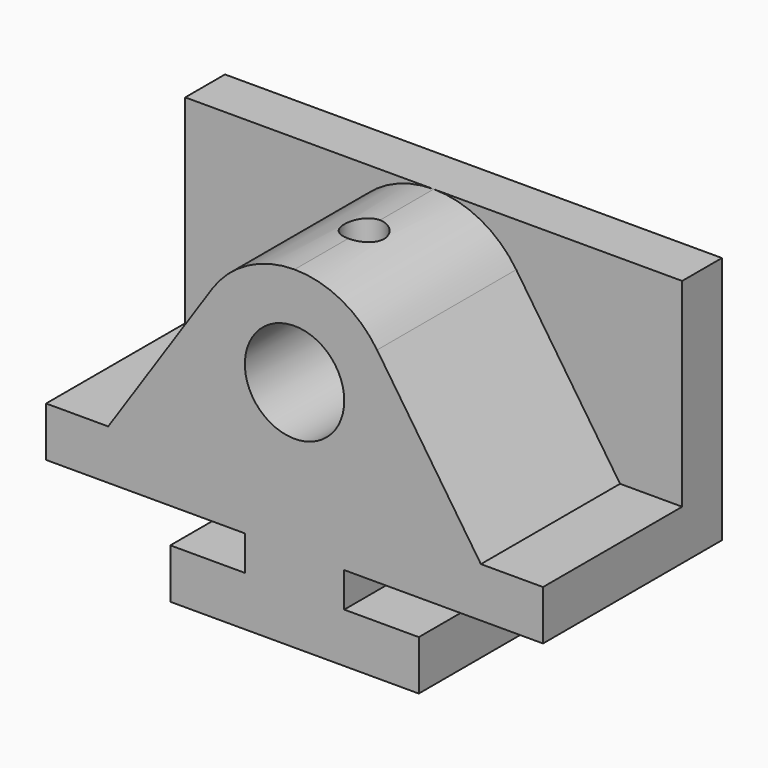
from build123d import *
from build123d import SkipClean  # not in build123d's __all__

# Parameters (mm, degrees)
F0_W     = 127
F0_H     = 85.09
F1_DEPTH = 57.15
F3_DEPTH = 57.151
F4_DEPTH = 44.45
F5_R     = 12.7
F6_DEPTH = 44.45
F7_R     = 5.08
F8_DEPTH = 13.7612578348


with BuildPart() as f1:
    # F0 (on Front) → F1 (new body)
    with BuildSketch(Plane.XZ):
        with Locations((63.5, 42.545)):
            Rectangle(F0_W, F0_H)
    extrude(amount=F1_DEPTH)

    # F2 (on face) → F3 (cut, through all)
    with BuildSketch(Plane.XZ.offset(57.15)):
        Polygon((0, 0), (31.75, 0), (31.75, 12.7), (50.8, 12.7), (50.8, 21.59), (0, 21.59), align=None)
        Polygon((95.25, 12.7), (95.25, 0), (127, 0), (127, 21.59), (76.2, 21.59), (76.2, 12.7), align=None)
    extrude(amount=-F3_DEPTH, mode=Mode.SUBTRACT)

    # F2 (on face) → F4 (cut)
    with BuildSketch(Plane.XZ.offset(57.15)):
        with BuildLine():
            Line((0, 85.09), (0, 34.29))
            Line((0, 34.29), (15.875, 34.29))
            Line((15.875, 34.29), (42.4065743945, 73.8401730104))
            ThreePointArc((42.4065743945, 73.8401730104), (51.5470588235, 82.1017647059), (63.5, 85.09))
            Line((63.5, 85.09), (0, 85.09))
        make_face()
        with BuildLine():
            Line((111.125, 34.29), (127, 34.29))
            Line((127, 34.29), (127, 85.09))
            Line((127, 85.09), (63.5, 85.09))
            ThreePointArc((63.5, 85.09), (75.4529411765, 82.1017647059), (84.5934256055, 73.8401730104))
            Line((84.5934256055, 73.8401730104), (111.125, 34.29))
        make_face()
    extrude(amount=-F4_DEPTH, mode=Mode.SUBTRACT)

    # F5 (on face) → F6 (cut)
    with BuildSketch(Plane.XZ.offset(57.15)):
        with Locations((63.5, 59.69)):
            Circle(F5_R)
    extrude(amount=-F6_DEPTH, mode=Mode.SUBTRACT)

    # F7 (on face) → F8 (cut, through all)
    with BuildSketch(Plane.XY.offset(85.09)):
        with Locations((63.5, -34.925)):
            Circle(F7_R)
    with SkipClean():  # cleaning this boolean's faces spoils the solid; the shape is the same uncleaned
        extrude(amount=-F8_DEPTH, mode=Mode.SUBTRACT)


solid = f1.part
